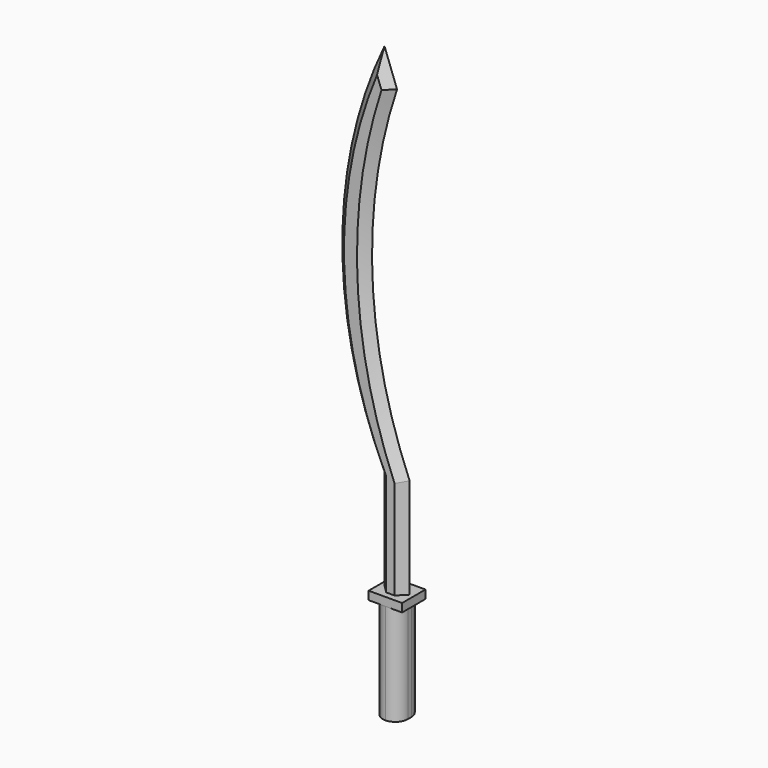
from build123d import *

# Parameters (mm, degrees)
F1_DEPTH = 44.45
F3_DEPTH = 44.45
F5_START = -9.525
F5_DEPTH = 25.4
F6_R     = 19.04999
F7_SIZE2 = 12.69999
F7_SIZE  = 12.69999


# Not quite as in the source:
# - a fillet or chamfer is up to 0.001 mm smaller than in the source, because OpenCascade refuses the exact size


with BuildPart() as f1:
    # F0 (on Front) → F1 (new body)
    with BuildSketch(Plane.XZ):
        Polygon((-19.05, -44.0120689886), (0, -44.0120689886), (19.05, -44.0120689886), (19.05, 108.3879310114), (-19.05, 108.3879310114), align=None)
    extrude(amount=F1_DEPTH)

    # F2 (on face) → F3 (join)
    with BuildSketch(Plane.XZ.offset(44.45)):
        Polygon((-25.4, 108.3879310114), (-19.05, 108.3879310114), (19.05, 108.3879310114), (25.4, 108.3879310114), (25.4, 121.0879310114), (-25.4, 121.0879310114), align=None)
    extrude(amount=-F3_DEPTH)

    # F4 (on face) → F5 (join)
    with BuildSketch(Plane.XZ.offset(44.45).offset(F5_START)):
        with BuildLine():
            Line((-19.05, 273.4879310114), (-19.05, 121.0879310114))
            Line((-19.05, 121.0879310114), (19.05, 121.0879310114))
            Line((19.05, 121.0879310114), (19.05, 273.4879310114))
            ThreePointArc((19.05, 273.4879310114), (-37.5025933071, 530.403553002), (0, 790.7828688622))
            Line((0, 790.7828688622), (-19.05, 842.4347043037))
            ThreePointArc((-19.05, 842.4347043037), (-83.1207001827, 557.9613176576), (-19.05, 273.4879310114))
        make_face()
    extrude(amount=-F5_DEPTH)

    # F6 (radius 19.05 in the source; OpenCascade refuses exactly that, so slightly less here)
    f6_edges = [f1.edges().sort_by_distance(p)[0] for p in [
        (19.05, 0, 32.187931),
        (19.05, -44.45, 32.187931),
        (-19.05, -44.45, 32.187931),
        (-19.05, 0, 32.187931),
    ]]
    fillet(f6_edges, radius=F6_R)

    # F7 (size 12.7 and 12.7 in the source; OpenCascade refuses exactly that, so slightly less here)
    f7_edges = [f1.edges().sort_by_distance(p)[0] for p in [
        (-37.502593, -34.925, 530.403553),
        (-37.502593, -9.525, 530.403553),
        (-83.1207, -34.925, 557.961318),
        (-83.1207, -9.525, 557.961318),
        (-9.525, -34.925, 816.608787),
        (-9.525, -9.525, 816.608787),
        (-19.05, -34.925, 197.287931),
        (-19.05, -9.525, 197.287931),
        (19.05, -34.925, 197.287931),
        (19.05, -9.525, 197.287931),
    ]]
    chamfer(f7_edges, length=F7_SIZE, length2=F7_SIZE2)


solid = f1.part
